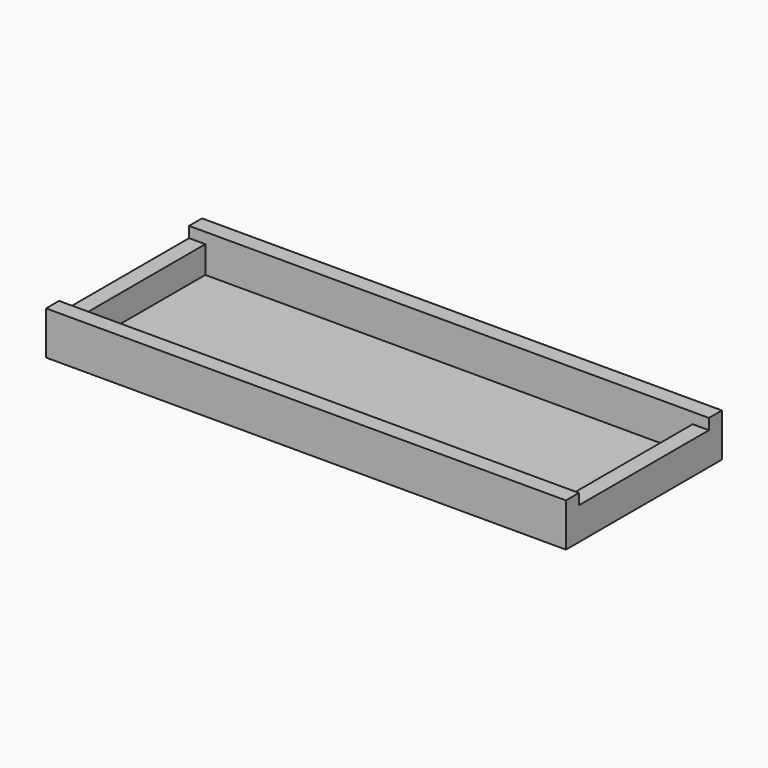
from build123d import *

# Parameters (mm, degrees)
F0_W     = 1219.2
F0_H     = 457.2
F1_DEPTH = 12.7
F2_W     = 1219.2
F2_H     = 38.1
F3_DEPTH = 88.9
F4_W     = 38.1
F4_H     = 381
F5_DEPTH = 63.5


# Not quite as in the source:
# - a length typed as a fraction of an inch, garbled in the dataset ("3 / 203.2 mm" for 3/8 in), is restored


with BuildPart() as f1:
    # F0 (on Top) → F1 (new body)
    with BuildSketch(Plane.XY):
        Rectangle(F0_W, F0_H)
    extrude(amount=F1_DEPTH)

    # F2 (on face) → F3 (join)
    with BuildSketch(Plane.XY.offset(12.7)):
        with Locations((0, -209.55)):
            Rectangle(F2_W, F2_H)
        with Locations((0, 209.55)):
            Rectangle(F2_W, F2_H)
    extrude(amount=F3_DEPTH)

    # F4 (on face) → F5 (join)
    with BuildSketch(Plane.XY.offset(12.7)):
        with Locations((-590.55, 0)):
            Rectangle(F4_W, F4_H)
        with Locations((590.55, 0)):
            Rectangle(F4_W, F4_H)
    extrude(amount=F5_DEPTH)


solid = f1.part
